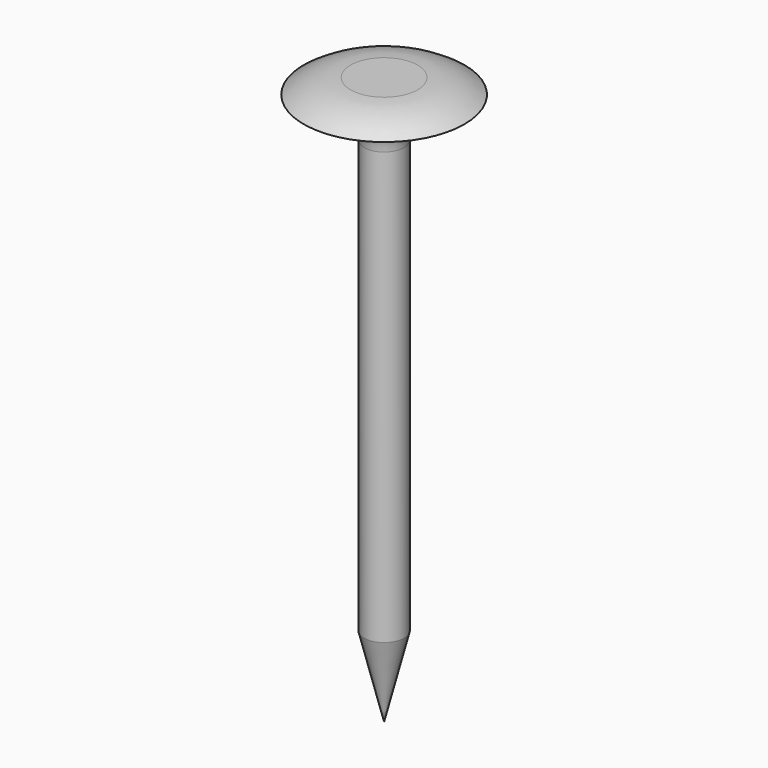
from build123d import *

# Parameters (mm, degrees)
F0_W     = 2.54
F0_H     = 69.85
F2_SIZE2 = 2.54
F2_SIZE  = 10.16
F3_R     = 5.08


# Not quite as in the source:
# - a fillet or chamfer that OpenCascade refuses, or shapes differently, is made with other operations: its cross-section is extruded or revolved along the edge and cut away or added


with BuildPart() as f1:
    # F0 (on Front) → F1 (revolve)
    with BuildSketch(Plane.XZ):
        Polygon((0, 14.605), (0, 12.7), (2.54, 12.7), (10.16, 12.7), (10.16, 14.605), align=None)
        with Locations((1.27, -22.225)):
            Rectangle(F0_W, F0_H)
    revolve(axis=Axis((0, 0, -22.225), (0, 0, -1)))

    # F2
    f2_edges = [f1.edges().sort_by_distance(p)[0] for p in [
        (-2.54, 0, -57.15),
    ]]
    f2_side = f1.faces().sort_by_distance((-2.54, 0, -22.225))[0]
    chamfer(f2_edges, length=F2_SIZE, length2=F2_SIZE2, reference=f2_side)

    # F3
    f3_edges = [f1.edges().sort_by_distance(p)[0] for p in [
        (-2.54, 0, 12.7),
    ]]
    fillet(f3_edges, radius=F3_R)

    # F4: fillet of radius 10.16 on 1 edges, made by hand

    # F4_s1 → F4_t2 (revolve, cut)
    with BuildSketch(Plane.XZ):
        with BuildLine():
            ThreePointArc((10.16, 12.7), (7.3479662746, 14.1170318444), (4.2371143013, 14.605))
            Line((4.2371143013, 14.605), (10.16, 14.605))
            Line((10.16, 14.605), (10.16, 12.7))
        make_face()
    revolve(axis=Axis((0, 0, 14.605), (0, 0, -1)), mode=Mode.SUBTRACT)


solid = f1.part
